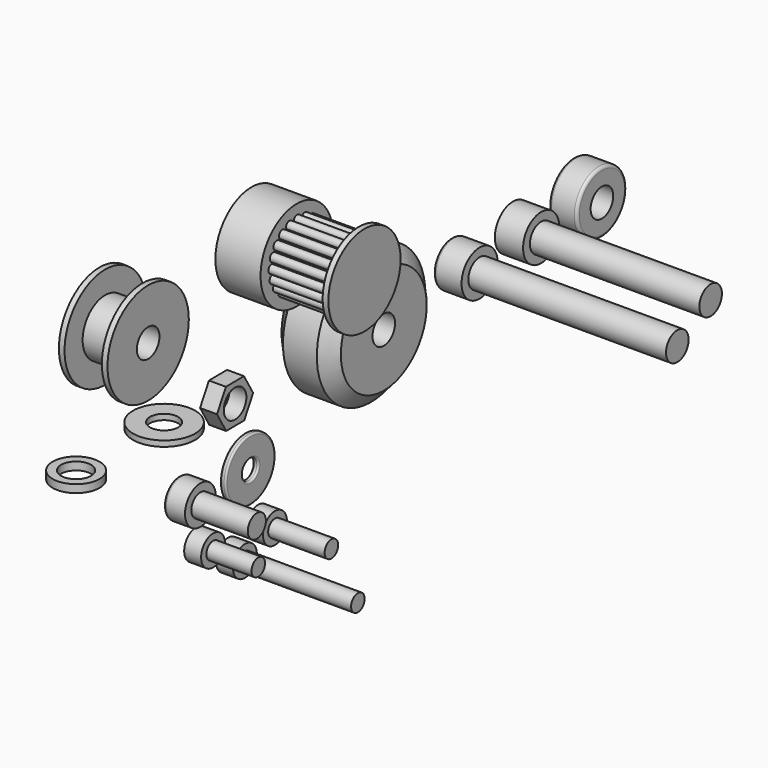
from build123d import *

# Parameters (mm, degrees)
F3_R      = 4
F4_DEPTH  = 5
F5_R      = 2.5
F6_DEPTH  = 30
F8_DEPTH  = 4
F9_R      = 5.5
F9_R_2    = 2.5
F10_DEPTH = 5
F11_R     = 0.5
F12_R     = 2.5
F13_DEPTH = 3
F14_R     = 5.5
F14_R_2   = 2.5
F15_DEPTH = 1
F16_R     = 4.15
F16_R_2   = 2.65
F17_DEPTH = 1.4
F18_R     = 3.4
F19_DEPTH = 3.8
F20_R     = 0.5
F22_DEPTH = 3
F23_R     = 2
F24_DEPTH = 10
F25_R     = 8
F26_DEPTH = 20
F28_R     = 8.8541204016
F28_R_2   = 5.5
F29_DEPTH = 11
F31_DEPTH = 12
F32_R     = 2.5
F33_DEPTH = 19
F34_R     = 4
F35_DEPTH = 5
F36_R     = 2.5
F37_DEPTH = 35
F38_R     = 0.5
F40_DEPTH = 4
F41_R     = 9
F41_R_2   = 2.5
F42_DEPTH = 8.6
F44_R     = 10.2643308429
F44_R_2   = 5
F45_DEPTH = 6.6
F46_R     = 2.65
F47_DEPTH = 3
F48_R     = 1.5
F49_DEPTH = 10
F51_DEPTH = 2
F52_R     = 2.65
F53_DEPTH = 3
F54_R     = 1.5
F55_DEPTH = 8
F57_DEPTH = 2
F58_R     = 2.65
F59_DEPTH = 3
F60_R     = 1.5
F61_DEPTH = 20
F63_DEPTH = 2
F64_R     = 5.5
F64_R_2   = 1.75
F65_DEPTH = 1
F66_R     = 0.3


with BuildPart() as f2:
    # F0 (on Top) → F2 (revolve)
    with BuildSketch(Plane.XY):
        Polygon((3, 12), (0, 12), (0, 2.5), (5.25, 2.5), (5.25, 9.5), align=None)
        Polygon((0, 2.5), (0, 12), (-3, 12), (-5.25, 9.5), (-5.25, 2.5), align=None)
    revolve(axis=Axis((-1.1980342679, 0, 0), (-1, 0, 0)))


with BuildPart() as f4:
    # F3 (on Right) → F4 (new body)
    with BuildSketch(Plane.YZ):
        with Locations((35.1446674716, 0)):
            Circle(F3_R)
    extrude(amount=F4_DEPTH)

    # F5 (on face) → F6 (join)
    with BuildSketch(Plane.YZ.offset(5)):
        with Locations((35.1446674716, 0)):
            Circle(F5_R)
    extrude(amount=F6_DEPTH)

    # F7 (on face) → F8 (cut)
    with BuildSketch(Plane(origin=(0, 0, 0), x_dir=(0, -1, 0), z_dir=(-1, 0, 0))):
        Polygon((-36.8588736636, -2.1569086285), (-34.1338329017, -2.5630004238), (-32.4196267097, -0.4060917954), (-33.4304612796, 2.1569086285), (-36.1555020415, 2.5630004238), (-37.8697082335, 0.4060917954), align=None)
    extrude(amount=-F8_DEPTH, mode=Mode.SUBTRACT)


with BuildPart() as f10:
    # F9 (on Right) → F10 (new body)
    with BuildSketch(Plane.YZ):
        with Locations((48.5870018601, 0)):
            Circle(F9_R)
        with Locations((48.5870018601, 0)):
            Circle(F9_R_2, mode=Mode.SUBTRACT)
    extrude(amount=F10_DEPTH)

    # F11
    f11_edges = [f10.edges().sort_by_distance(p)[0] for p in [
        (5, 43.087002, 0),
        (0, 43.087002, 0),
    ]]
    fillet(f11_edges, radius=F11_R)


with BuildPart() as f13:
    # F12 (on Right) → F13 (new body)
    with BuildSketch(Plane.YZ):
        Polygon((-32.0650244918, -3.4815789249), (-28.0651795794, -3.4463556858), (-26.095761343, 0.0352232391), (-28.1261880191, 3.4815789249), (-32.1260329315, 3.4463556858), (-34.0954511679, -0.0352232391), align=None)
        with Locations((-30.0956062554, 0)):
            Circle(F12_R, mode=Mode.SUBTRACT)
    extrude(amount=F13_DEPTH)


with BuildPart() as f15:
    # F14 (on Top) → F15 (new body)
    with BuildSketch(Plane.XY):
        with Locations((0, -42.0582406223)):
            Circle(F14_R)
        with Locations((0, -42.0582406223)):
            Circle(F14_R_2, mode=Mode.SUBTRACT)
    extrude(amount=F15_DEPTH)


with BuildPart() as f17:
    # F16 (on Top) → F17 (new body)
    with BuildSketch(Plane.XY):
        with Locations((0, -61.5273416042)):
            Circle(F16_R)
        with Locations((0, -61.5273416042)):
            Circle(F16_R_2, mode=Mode.SUBTRACT)
    extrude(amount=F17_DEPTH)


with BuildPart() as f19:
    # F18 (on Right) → F19 (new body)
    with BuildSketch(Plane.YZ):
        with Locations((-38.7737825513, -12.0268082246)):
            Circle(F18_R)
    extrude(amount=F19_DEPTH)

    # F20
    f20_edges = [f19.edges().sort_by_distance(p)[0] for p in [
        (0, -42.173783, -12.026808),
    ]]
    fillet(f20_edges, radius=F20_R)

    # F21 (on face) → F22 (cut)
    with BuildSketch(Plane(origin=(0, 0, 0), x_dir=(0, -1, 0), z_dir=(-1, 0, 0))):
        Polygon((37.9488725525, -10.2452280877), (36.8184338945, -11.8504111709), (37.6433438932, -13.6319913078), (39.59869255, -13.8083883615), (40.7291312081, -12.2032052783), (39.9042212094, -10.4216251414), align=None)
    extrude(amount=-F22_DEPTH, mode=Mode.SUBTRACT)

    # F23 (on face) → F24 (join)
    with BuildSketch(Plane.YZ.offset(3.8)):
        with Locations((-38.7737825513, -12.0268082246)):
            Circle(F23_R)
    extrude(amount=F24_DEPTH)


with BuildPart() as f26:
    # F25 (on Right) → F26 (new body)
    with BuildSketch(Plane.YZ):
        with Locations((-22.7080509067, 21.7676777393)):
            Circle(F25_R)
    extrude(amount=F26_DEPTH)

    # F28 (on offset) → F29 (cut)
    with BuildSketch(Plane.YZ.offset(19)):
        with Locations((-22.7080509067, 21.7676777393)):
            Circle(F28_R)
        with Locations((-22.7080509067, 21.7676777393)):
            Circle(F28_R_2, mode=Mode.SUBTRACT)
    extrude(amount=-F29_DEPTH, mode=Mode.SUBTRACT)

    # F30 (on face) → F31 (join, through all)
    with BuildSketch(Plane.YZ.offset(8)):
        with BuildLine():
            ThreePointArc((-28.1691927708, 21.1150449637), (-27.6636023002, 21.3473653709), (-27.4572059699, 21.8640810087))
            ThreePointArc((-27.4572059699, 21.8640810087), (-27.6546288882, 22.3711890532), (-28.1429621534, 22.6113244309))
            ThreePointArc((-28.1429621534, 22.6113244309), (-28.2072059699, 21.8640810087), (-28.1691927708, 21.1150449637))
        make_face()
        with BuildLine():
            ThreePointArc((-28.1691927708, 21.1150449637), (-28.2072059699, 21.8640810087), (-28.1429621534, 22.6113244309))
            ThreePointArc((-28.1429621534, 22.6113244309), (-28.9570907513, 21.877226909), (-28.1691927708, 21.1150449637))
        make_face()
        with BuildLine():
            ThreePointArc((-27.6162574984, 24.2495133609), (-27.9082679151, 23.5586950661), (-28.1035800817, 22.83457273))
            ThreePointArc((-28.1035800817, 22.83457273), (-27.4521890431, 22.963302706), (-27.1582679151, 23.5586950661))
            ThreePointArc((-27.1582679151, 23.5586950661), (-27.2831647986, 23.9731176689), (-27.6162574984, 24.2495133609))
        make_face()
        with BuildLine():
            ThreePointArc((-27.6162574984, 24.2495133609), (-28.6173884163, 23.8029247015), (-28.1035800817, 22.83457273))
            ThreePointArc((-28.1035800817, 22.83457273), (-27.9082679151, 23.5586950661), (-27.6162574984, 24.2495133609))
        make_face()
        with BuildLine():
            ThreePointArc((-27.7002308442, 19.4594014406), (-27.9678484122, 20.1600303276), (-28.1376598283, 20.8905534846))
            ThreePointArc((-28.1376598283, 20.8905534846), (-28.6850935266, 19.9408056805), (-27.7002308442, 19.4594014406))
        make_face()
        with BuildLine():
            ThreePointArc((-27.2178484122, 20.1600303276), (-27.501403647, 20.7473371307), (-28.1376598283, 20.8905534846))
            ThreePointArc((-28.1376598283, 20.8905534846), (-27.9678484122, 20.1600303276), (-27.7002308442, 19.4594014406))
            ThreePointArc((-27.7002308442, 19.4594014406), (-27.3501052714, 19.734714666), (-27.2178484122, 20.1600303276))
        make_face()
        with BuildLine():
            ThreePointArc((-26.6091033847, 25.6447629284), (-27.1002963875, 25.0779918688), (-27.5098154041, 24.4496653811))
            ThreePointArc((-27.5098154041, 24.4496653811), (-26.7429724885, 24.4185833222), (-26.3502963875, 25.0779918688))
            ThreePointArc((-26.3502963875, 25.0779918688), (-26.4180593495, 25.38952457), (-26.6091033847, 25.6447629284))
        make_face()
        with BuildLine():
            ThreePointArc((-26.6091033847, 25.6447629284), (-27.6992389531, 25.529398341), (-27.5098154041, 24.4496653811))
            ThreePointArc((-27.5098154041, 24.4496653811), (-27.1002963875, 25.0779918688), (-26.6091033847, 25.6447629284))
        make_face()
        with BuildLine():
            ThreePointArc((-26.7425995628, 18.0297080843), (-27.2136252276, 18.6133473763), (-27.6008695516, 19.2556415717))
            ThreePointArc((-27.6008695516, 19.2556415717), (-27.8280217259, 18.1832114177), (-26.7425995628, 18.0297080843))
        make_face()
        with BuildLine():
            ThreePointArc((-25.2200870742, 26.6604963843), (-25.8623812696, 26.2732520602), (-26.4460205616, 25.8022263954))
            ThreePointArc((-26.4460205616, 25.8022263954), (-25.612610844, 25.5660641541), (-25.1123812696, 26.2732520602))
            ThreePointArc((-25.1123812696, 26.2732520602), (-25.1398092502, 26.4742238908), (-25.2200870742, 26.6604963843))
        make_face()
        with BuildLine():
            ThreePointArc((-25.2200870742, 26.6604963843), (-26.2925172282, 26.8876485585), (-26.4460205616, 25.8022263954))
            ThreePointArc((-26.4460205616, 25.8022263954), (-25.8623812696, 26.2732520602), (-25.2200870742, 26.6604963843))
        make_face()
        with BuildLine():
            ThreePointArc((-25.3900385485, 16.9659132418), (-26.0183650362, 17.3754322584), (-26.5851360958, 17.8666252612))
            ThreePointArc((-26.5851360958, 17.8666252612), (-26.4697715084, 16.7764896928), (-25.3900385485, 16.9659132418))
        make_face()
        with BuildLine():
            ThreePointArc((-23.5851751613, 27.1972866609), (-24.3156983184, 27.0274752448), (-25.0163272053, 26.7598576768))
            ThreePointArc((-25.0163272053, 26.7598576768), (-24.1796315429, 26.2899212925), (-23.5656983184, 27.0274752448))
            ThreePointArc((-23.5656983184, 27.0274752448), (-23.5705834387, 27.1129376115), (-23.5851751613, 27.1972866609))
        make_face()
        with BuildLine():
            ThreePointArc((-23.5851751613, 27.1972866609), (-24.5349229654, 27.7447203592), (-25.0163272053, 26.7598576768))
            ThreePointArc((-25.0163272053, 26.7598576768), (-24.3156983184, 27.0274752448), (-23.5851751613, 27.1972866609))
        make_face()
        with BuildLine():
            ThreePointArc((-23.7749458974, 16.3721485642), (-24.4990682335, 16.5674607308), (-25.1898865283, 16.8594711475))
            ThreePointArc((-25.1898865283, 16.8594711475), (-24.7432978689, 15.8583402296), (-23.7749458974, 16.3721485642))
        make_face()
        with BuildLine():
            ThreePointArc((-21.864404215, 27.202588986), (-22.6116476373, 27.2668328025), (-23.3606836822, 27.2288196034))
            ThreePointArc((-23.3606836822, 27.2288196034), (-22.6247935376, 26.5169480212), (-21.864404215, 27.202588986))
        make_face()
        with BuildLine():
            ThreePointArc((-21.8616476373, 27.2668328025), (-22.6306603469, 28.016591775), (-23.3606836822, 27.2288196034))
            ThreePointArc((-23.3606836822, 27.2288196034), (-22.6116476373, 27.2668328025), (-21.864404215, 27.202588986))
            ThreePointArc((-21.864404215, 27.202588986), (-21.8623370986, 27.234681338), (-21.8616476373, 27.2668328025))
        make_face()
        with BuildLine():
            ThreePointArc((-22.0554181311, 16.3065358751), (-22.8044541761, 16.268522676), (-23.5516975983, 16.3327664925))
            ThreePointArc((-23.5516975983, 16.3327664925), (-22.8366056406, 15.5192121374), (-22.0544541761, 16.268522676))
            ThreePointArc((-22.0544541761, 16.268522676), (-22.0546952035, 16.2875353857), (-22.0554181311, 16.3065358751))
        make_face()
        with BuildLine():
            ThreePointArc((-20.226215285, 26.675884331), (-20.9170335799, 26.9678947477), (-21.6411559159, 27.1632069143))
            ThreePointArc((-21.6411559159, 27.1632069143), (-21.1612632153, 26.2587742466), (-20.226215285, 26.675884331))
        make_face()
        with BuildLine():
            ThreePointArc((-20.1670335799, 26.9678947477), (-20.8185240677, 27.7113971862), (-21.6411559159, 27.1632069143))
            ThreePointArc((-21.6411559159, 27.1632069143), (-20.9170335799, 26.9678947477), (-20.226215285, 26.675884331))
            ThreePointArc((-20.226215285, 26.675884331), (-20.1819778945, 26.8189211278), (-20.1670335799, 26.9678947477))
        make_face()
        with BuildLine():
            ThreePointArc((-20.399774608, 16.7754978017), (-21.100403495, 16.5078802337), (-21.830926652, 16.3380688176))
            ThreePointArc((-21.830926652, 16.3380688176), (-21.0149411283, 15.762765354), (-20.350403495, 16.5078802337))
            ThreePointArc((-20.350403495, 16.5078802337), (-20.3628495426, 16.6439470091), (-20.399774608, 16.7754978017))
        make_face()
        with BuildLine():
            ThreePointArc((-18.8309657176, 25.6687302173), (-19.3977367772, 26.1599232201), (-20.0260632648, 26.5694422367))
            ThreePointArc((-20.0260632648, 26.5694422367), (-19.8491432494, 25.5609806545), (-18.8309657176, 25.6687302173))
        make_face()
        with BuildLine():
            ThreePointArc((-18.6477367772, 26.1599232201), (-19.1841306744, 26.878861627), (-20.0260632648, 26.5694422367))
            ThreePointArc((-20.0260632648, 26.5694422367), (-19.3977367772, 26.1599232201), (-18.8309657176, 25.6687302173))
            ThreePointArc((-18.8309657176, 25.6687302173), (-18.6950354556, 25.8977956698), (-18.6477367772, 26.1599232201))
        make_face()
        with BuildLine():
            ThreePointArc((-18.9700812517, 17.7331290831), (-19.5537205437, 17.2621034184), (-20.1960147391, 16.8748590943))
            ThreePointArc((-20.1960147391, 16.8748590943), (-19.352748713, 16.5395313989), (-18.8037205437, 17.2621034184))
            ThreePointArc((-18.8037205437, 17.2621034184), (-18.8465326376, 17.511873844), (-18.9700812517, 17.7331290831))
        make_face()
        with BuildLine():
            ThreePointArc((-17.8152322617, 24.2797139068), (-18.2024765858, 24.9220081023), (-18.6735022505, 25.5056473942))
            ThreePointArc((-18.6735022505, 25.5056473942), (-18.8168730841, 24.4918721437), (-17.8152322617, 24.2797139068))
        make_face()
        with BuildLine():
            ThreePointArc((-17.4524765858, 24.9220081023), (-17.8790335835, 25.5986798279), (-18.6735022505, 25.5056473942))
            ThreePointArc((-18.6735022505, 25.5056473942), (-18.2024765858, 24.9220081023), (-17.8152322617, 24.2797139068))
            ThreePointArc((-17.8152322617, 24.2797139068), (-17.5494324666, 24.5531810717), (-17.4524765858, 24.9220081023))
        make_face()
        with BuildLine():
            ThreePointArc((-17.9062864092, 19.0856900974), (-18.3158054258, 18.4573636098), (-18.8069984286, 17.8905925502))
            ThreePointArc((-18.8069984286, 17.8905925502), (-18.0042727246, 17.7751265717), (-17.5658054258, 18.4573636098))
            ThreePointArc((-17.5658054258, 18.4573636098), (-17.6563968793, 18.8146875087), (-17.9062864092, 19.0856900974))
        make_face()
        with BuildLine():
            ThreePointArc((-16.6982534011, 23.375325151), (-17.0229377395, 23.9930682918), (-17.7158709691, 24.0759540379))
            ThreePointArc((-17.7158709691, 24.0759540379), (-17.4482534011, 23.375325151), (-17.278441985, 22.6448019939))
            ThreePointArc((-17.278441985, 22.6448019939), (-16.8609465979, 22.9088803858), (-16.6982534011, 23.375325151))
        make_face()
        with BuildLine():
            ThreePointArc((-17.3125217316, 20.7007827485), (-17.5078338982, 19.9766604125), (-17.7998443149, 19.2858421176))
            ThreePointArc((-17.7998443149, 19.2858421176), (-17.0934112954, 19.3515572959), (-16.7578338982, 19.9766604125))
            ThreePointArc((-16.7578338982, 19.9766604125), (-16.9124415381, 20.4327392845), (-17.3125217316, 20.7007827485))
        make_face()
        with BuildLine():
            ThreePointArc((-17.2080509067, 21.7676777393), (-17.2177740351, 22.0945720244), (-17.2469090425, 22.4203105149))
            ThreePointArc((-17.2469090425, 22.4203105149), (-17.9587806248, 21.6844203702), (-17.2731396599, 20.9240310477))
            ThreePointArc((-17.2731396599, 20.9240310477), (-17.2243472377, 21.3446008296), (-17.2080509067, 21.7676777393))
        make_face()
        with BuildLine():
            ThreePointArc((-16.4588958434, 21.6712744699), (-16.6921802056, 22.2148781395), (-17.2469090425, 22.4203105149))
            ThreePointArc((-17.2469090425, 22.4203105149), (-17.2177740351, 22.0945720244), (-17.2080509067, 21.7676777393))
            ThreePointArc((-17.2080509067, 21.7676777393), (-17.2243472377, 21.3446008296), (-17.2731396599, 20.9240310477))
            ThreePointArc((-17.2731396599, 20.9240310477), (-16.7017877989, 21.1186973882), (-16.4588958434, 21.6712744699))
        make_face()
    extrude(amount=F31_DEPTH)

    # F32 (on face) → F33 (cut)
    with BuildSketch(Plane(origin=(0, 0, 0), x_dir=(0, -1, 0), z_dir=(-1, 0, 0))):
        with Locations((22.7080509067, 21.7676777393)):
            Circle(F32_R)
    extrude(amount=-F33_DEPTH, mode=Mode.SUBTRACT)


with BuildPart() as f35:
    # F34 (on Right) → F35 (new body)
    with BuildSketch(Plane.YZ):
        with Locations((21.5235669166, 0)):
            Circle(F34_R)
    extrude(amount=F35_DEPTH)

    # F36 (on face) → F37 (join)
    with BuildSketch(Plane.YZ.offset(5)):
        with Locations((21.5235669166, 0)):
            Circle(F36_R)
    extrude(amount=F37_DEPTH)

    # F38
    f38_edges = [f35.edges().sort_by_distance(p)[0] for p in [
        (0, 17.523567, 0),
    ]]
    fillet(f38_edges, radius=F38_R)

    # F39 (on face) → F40 (cut)
    with BuildSketch(Plane(origin=(0, 0, 0), x_dir=(0, -1, 0), z_dir=(-1, 0, 0))):
        Polygon((-23.9366982132, 1.3932220037), (-23.9366982132, -1.3932220037), (-21.5235669166, -2.7864440074), (-19.11043562, -1.3932220037), (-19.11043562, 1.3932220037), (-21.5235669166, 2.7864440074), align=None)
    extrude(amount=-F40_DEPTH, mode=Mode.SUBTRACT)


with BuildPart() as f42:
    # F41 (on Right) → F42 (new body)
    with BuildSketch(Plane.YZ):
        with Locations((-56.3313961029, 21.93595469)):
            Circle(F41_R)
        with Locations((-56.3313961029, 21.93595469)):
            Circle(F41_R_2, mode=Mode.SUBTRACT)
    extrude(amount=F42_DEPTH)

    # F44 (on offset) → F45 (cut)
    with BuildSketch(Plane.YZ.offset(7.6)):
        with Locations((-56.3313961029, 21.93595469)):
            Circle(F44_R)
        with Locations((-56.3313961029, 21.93595469)):
            Circle(F44_R_2, mode=Mode.SUBTRACT)
    extrude(amount=-F45_DEPTH, mode=Mode.SUBTRACT)


with BuildPart() as f47:
    # F46 (on Right) → F47 (new body)
    with BuildSketch(Plane.YZ):
        with Locations((-21.2763492018, -22.9839254171)):
            Circle(F46_R)
    extrude(amount=F47_DEPTH)

    # F48 (on face) → F49 (join)
    with BuildSketch(Plane.YZ.offset(3)):
        with Locations((-21.2763492018, -22.9839254171)):
            Circle(F48_R)
    extrude(amount=F49_DEPTH)

    # F50 (on face) → F51 (cut)
    with BuildSketch(Plane(origin=(0, 0, 0), x_dir=(0, -1, 0), z_dir=(-1, 0, 0))):
        Polygon((19.7282508016, -22.090130389), (19.7282508016, -23.8777204452), (21.2763492018, -24.7715154733), (22.824447602, -23.8777204452), (22.824447602, -22.090130389), (21.2763492018, -21.1963353609), align=None)
    extrude(amount=-F51_DEPTH, mode=Mode.SUBTRACT)


with BuildPart() as f53:
    # F52 (on Right) → F53 (new body)
    with BuildSketch(Plane.YZ):
        with Locations((-34.9578261375, -20.9107287228)):
            Circle(F52_R)
    extrude(amount=F53_DEPTH)

    # F54 (on face) → F55 (join)
    with BuildSketch(Plane.YZ.offset(3)):
        with Locations((-34.9578261375, -20.9107287228)):
            Circle(F54_R)
    extrude(amount=F55_DEPTH)

    # F56 (on face) → F57 (cut)
    with BuildSketch(Plane(origin=(0, 0, 0), x_dir=(0, -1, 0), z_dir=(-1, 0, 0))):
        Polygon((34.5067056588, -19.0262736238), (33.1002799102, -20.359182968), (33.5514003889, -22.243638067), (35.4089466162, -22.7951838218), (36.8153723649, -21.4622744776), (36.3642518862, -19.5778193786), align=None)
    extrude(amount=-F57_DEPTH, mode=Mode.SUBTRACT)


with BuildPart() as f59:
    # F58 (on Right) → F59 (new body)
    with BuildSketch(Plane.YZ):
        with Locations((-27.9216468334, -25.4082437605)):
            Circle(F58_R)
    extrude(amount=F59_DEPTH)

    # F60 (on face) → F61 (join)
    with BuildSketch(Plane.YZ.offset(3)):
        with Locations((-27.9216468334, -25.4082437605)):
            Circle(F60_R)
    extrude(amount=F61_DEPTH)

    # F62 (on face) → F63 (cut)
    with BuildSketch(Plane(origin=(0, 0, 0), x_dir=(0, -1, 0), z_dir=(-1, 0, 0))):
        Polygon((29.4106741131, -24.1658073834), (27.5901790082, -23.4974901208), (26.1011517284, -24.7399264978), (26.4326195537, -26.6506801375), (28.2531146587, -27.3189974002), (29.7421419384, -26.0765610231), align=None)
    extrude(amount=-F63_DEPTH, mode=Mode.SUBTRACT)


with BuildPart() as f65:
    # F64 (on Right) → F65 (new body)
    with BuildSketch(Plane.YZ):
        with Locations((-24.1639036685, -13.4048396721)):
            Circle(F64_R)
        with Locations((-24.1639036685, -13.4048396721)):
            Circle(F64_R_2, mode=Mode.SUBTRACT)
    extrude(amount=F65_DEPTH)

    # F66
    f66_edges = [f65.edges().sort_by_distance(p)[0] for p in [
        (1, -29.663904, -13.40484),
        (1, -25.913904, -13.40484),
        (0, -25.913904, -13.40484),
        (0, -29.663904, -13.40484),
    ]]
    fillet(f66_edges, radius=F66_R)


solid = Compound([f2.part, f4.part, f10.part, f13.part, f15.part, f17.part, f19.part, f26.part, f35.part, f42.part, f47.part, f53.part, f59.part, f65.part])
